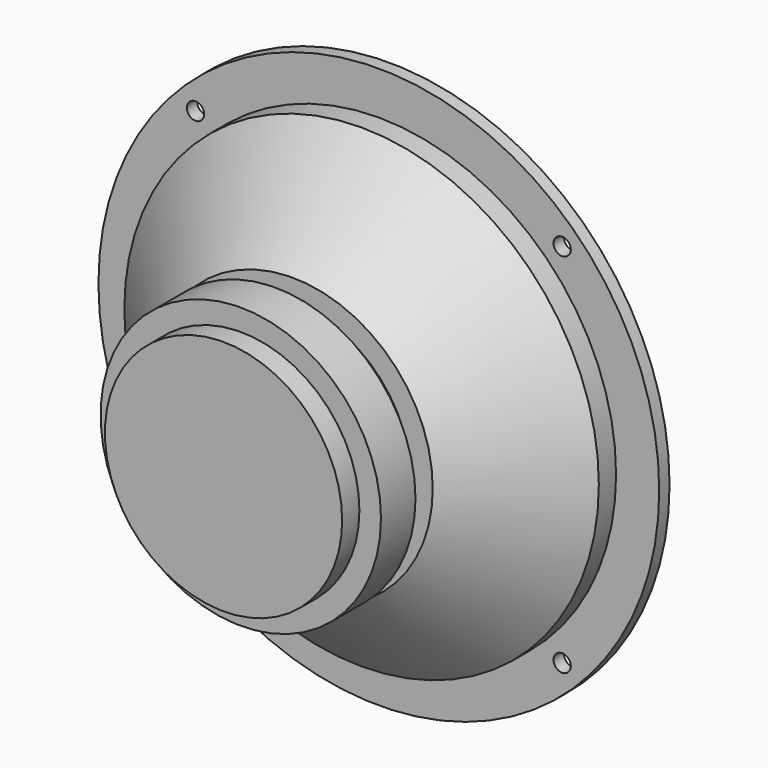
from build123d import *

# Parameters (mm, degrees)
F0_R      = 55
F1_DEPTH  = 25
F2_SIZE2  = 20
F2_SIZE   = 22.5
F3_R      = 27.5
F4_DEPTH  = 20
F6_START  = -5
F5_R      = 32.5
F5_R_2    = 27.5
F6_DEPTH  = 10
F7_R      = 65
F8_DEPTH  = 3
F9_R      = 2
F10_DEPTH = 25
F11_R     = 45
F12_DEPTH = 15
F12_TAPER = 60
F13_DEPTH = 10
F15_R     = 55
F15_R_2   = 45
F16_DEPTH = 4


# Not quite as in the source:
# - a fillet or chamfer that OpenCascade refuses, or shapes differently, is made with other operations: its cross-section is extruded or revolved along the edge and cut away or added


with BuildPart() as f1:
    # F0 (on Front) → F1 (new body)
    with BuildSketch(Plane.XZ):
        Circle(F0_R)
    extrude(amount=F1_DEPTH)

    # F2
    f2_edges = [f1.edges().sort_by_distance(p)[0] for p in [
        (-55, -25, 0),
    ]]
    f2_side = f1.faces().sort_by_distance((0, -25, 0))[0]
    chamfer(f2_edges, length=F2_SIZE, length2=F2_SIZE2, reference=f2_side)

    # F3 (on face) → F4 (join)
    with BuildSketch(Plane.XZ.offset(25)):
        Circle(F3_R)
    extrude(amount=F4_DEPTH)

    # F5 (on face) → F6 (join)
    with BuildSketch(Plane.XZ.offset(45).offset(F6_START)):
        Circle(F5_R)
        Circle(F5_R_2, mode=Mode.SUBTRACT)
    extrude(amount=-F6_DEPTH)

    # F7 (on face) → F8 (join)
    with BuildSketch(Plane(origin=(0, 0, 0), x_dir=(-1, 0, 0), z_dir=(0, 1, 0))):
        Circle(F7_R)
    extrude(amount=F8_DEPTH)

    # F9 (on face) → F10 (cut)
    with BuildSketch(Plane(origin=(0, 3, 0), x_dir=(-1, 0, 0), z_dir=(0, 1, 0))):
        with Locations((-42.5, 42.5)):
            Circle(F9_R)
        with Locations((42.5, 42.5)):
            Circle(F9_R)
        with Locations((42.5, -42.5)):
            Circle(F9_R)
        with Locations((-42.5, -42.5)):
            Circle(F9_R)
    extrude(amount=-F10_DEPTH, mode=Mode.SUBTRACT)

    # F11 (on face) → F12 (cut)
    with BuildSketch(Plane(origin=(0, 3, 0), x_dir=(-1, 0, 0), z_dir=(0, 1, 0))):
        Circle(F11_R)
    extrude(amount=-F12_DEPTH, taper=F12_TAPER, mode=Mode.SUBTRACT)

    # F13 (add): a face of the model
    f13_faces = [f1.faces().sort_by_distance(p)[0] for p in [
        (0, -12, 0),
    ]]
    extrude(f13_faces, amount=F13_DEPTH)

    # F14: fillet of radius 23 on 1 edges, made by hand

    # F14_s1 → F14_t2 (revolve, cut)
    with BuildSketch(Plane.XY):
        with BuildLine():
            ThreePointArc((-19.0192378865, -12), (-10.7693772202, -4.6530100506), (-0.0455719255, -2))
            Line((-0.0455719255, -2), (-19.0192378865, -2))
            Line((-19.0192378865, -2), (-19.0192378865, -12))
        make_face()
    revolve(axis=Axis((0, -2, 0), (0, 1, 0)), mode=Mode.SUBTRACT)

    # F15 (on face) → F16 (join)
    with BuildSketch(Plane(origin=(0, 3, 0), x_dir=(-1, 0, 0), z_dir=(0, 1, 0))):
        Circle(F15_R)
        Circle(F15_R_2, mode=Mode.SUBTRACT)
    extrude(amount=F16_DEPTH)

    # F17: fillet of radius 5.1 on 2 edges, made by hand

    # F17_s1 → F17_t2 (revolve, cut)
    with BuildSketch(Plane.XY):
        with BuildLine():
            ThreePointArc((-55, 3), (-53.2137840453, 5.8761790704), (-50.0200401608, 7))
            Line((-50.0200401608, 7), (-55, 7))
            Line((-55, 7), (-55, 3))
        make_face()
    revolve(axis=Axis((0, 7, 0), (0, 1, 0)), mode=Mode.SUBTRACT)

    # F17_s3 → F17_t4 (revolve, cut)
    with BuildSketch(Plane.XY):
        with BuildLine():
            ThreePointArc((-49.9799598392, 7), (-46.7862159547, 5.8761790704), (-45, 3))
            Line((-45, 3), (-45, 7))
            Line((-45, 7), (-49.9799598392, 7))
        make_face()
    revolve(axis=Axis((0, 7, 0), (0, 1, 0)), mode=Mode.SUBTRACT)


solid = f1.part
